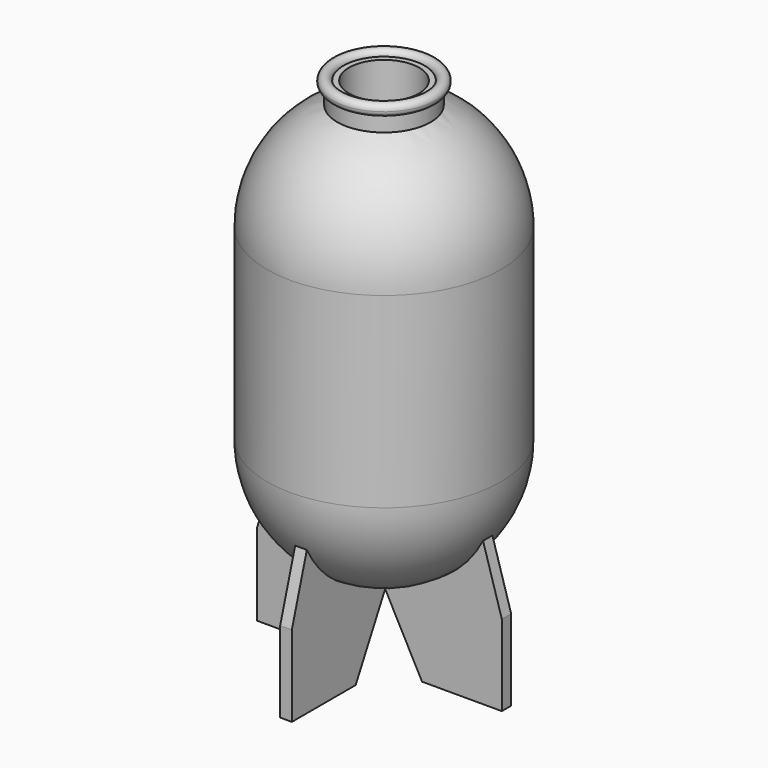
from build123d import *

# Parameters (mm, degrees)
F0_R      = 31.75
F0_R_2    = 28.575
F1_DEPTH  = 25.4
F3_ANGLE  = 180
F6_R      = 12.7
F7_DEPTH  = 3.175
F8_R      = 9.525
F9_DEPTH  = 25.4
F11_DEPTH = 1.5875
F13_COUNT = 4
F13_ANGLE = 270
F14_R     = 1.5875


with BuildPart() as f1:
    # F0 (on Top) → F1 (new body, symmetric)
    with BuildSketch(Plane.XY):
        Circle(F0_R)
        Circle(F0_R_2, mode=Mode.SUBTRACT)
    extrude(amount=F1_DEPTH, both=True)

    # F2 (on face) → F3 (revolve)
    with BuildSketch(Plane.XY.offset(25.4)):
        with BuildLine():
            Line((0, -25.4), (0, -31.75))
            ThreePointArc((0, -31.75), (31.75, 0), (0, 31.75))
            Line((0, 31.75), (0, 25.4))
            ThreePointArc((0, 25.4), (25.4, 0), (0, -25.4))
        make_face()
    revolve(axis=Axis((0, 0, 25.4), (0, -1, 0)), revolution_arc=F3_ANGLE)

    # F4: F1 across plane


with BuildPart() as f1_1:
    add(f1.part)
    add(f1.part.mirror(Plane.XY))

    # F6 (on offset) → F7 (join, symmetric)
    with BuildSketch(Plane.XY.offset(57.15)):
        Circle(F6_R)
    extrude(amount=F7_DEPTH, both=True)

    # F8 (on face) → F9 (cut)
    with BuildSketch(Plane.XY.offset(60.325)):
        Circle(F8_R)
    extrude(amount=-F9_DEPTH, mode=Mode.SUBTRACT)

    # F14 (on Front) → F15 (revolve)
    with BuildSketch(Plane.XZ):
        with Locations((12.5909885392, 60.2298639715)):
            Circle(F14_R)
    revolve(axis=Axis((0, 0, 39.1259763025), (0, 0, -1)))


with BuildPart() as f11:
    # F10 (on Front) → F11 (new body, symmetric)
    with BuildSketch(Plane.XZ):
        with BuildLine():
            ThreePointArc((28.195271218, -39.9975744884), (16.5013561563, -52.5250390784), (0, -57.15))
            Line((0, -57.15), (11.6054198963, -79.0879651904))
            Line((11.6054198963, -79.0879651904), (33.2879051566, -79.0879651904))
            Line((33.2879051566, -79.0879651904), (33.2879051566, -57.0490099723))
            Line((33.2879051566, -57.0490099723), (28.195271218, -39.9975744884))
        make_face()
    extrude(amount=F11_DEPTH, both=True)


with BuildPart() as f13_1:
    # F13: instance of F11
    add(f11.part.rotate(Axis((0, 0, 1.7845220864), (0, 0, -1)), 1 * F13_ANGLE / (F13_COUNT - 1)))


with BuildPart() as f13_2:
    # F13: instance of F11
    add(f11.part.rotate(Axis((0, 0, 1.7845220864), (0, 0, -1)), 2 * F13_ANGLE / (F13_COUNT - 1)))


with BuildPart() as f13_3:
    # F13: instance of F11
    add(f11.part.rotate(Axis((0, 0, 1.7845220864), (0, 0, -1)), 3 * F13_ANGLE / (F13_COUNT - 1)))


solid = Compound([f1_1.part, f11.part, f13_1.part, f13_2.part, f13_3.part])
